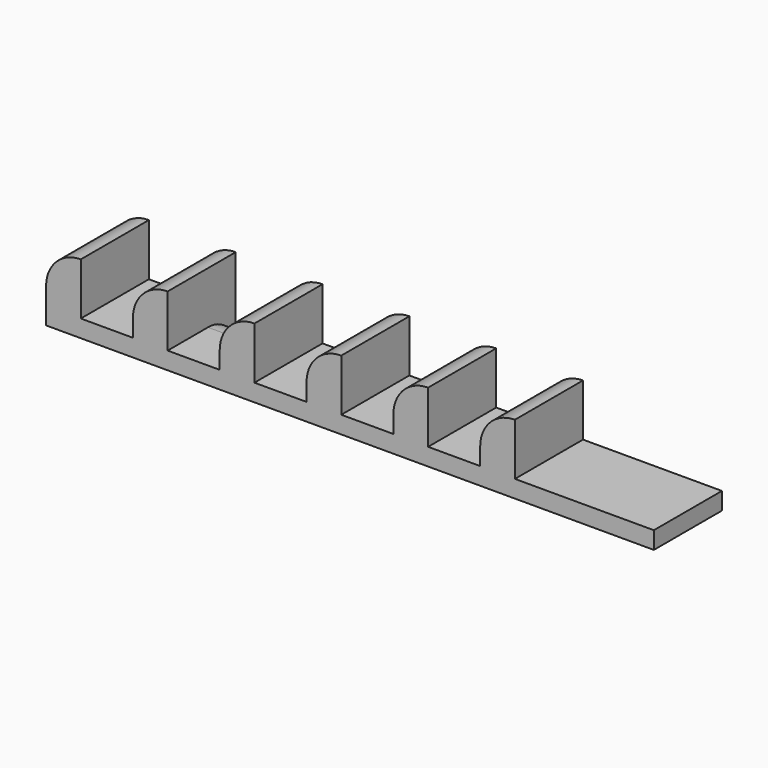
from build123d import *

# Parameters (mm, degrees)
F0_W        = 88.9
F0_H        = 12.446
F1_DEPTH    = 2.54
F2_W        = 5.08
F2_H        = 12.446
F3_DEPTH    = 7.62
F4_T1_DEPTH = 37.846
F4_T3_DEPTH = 7.62


# Not quite as in the source:
# - a fillet or chamfer that OpenCascade refuses, or shapes differently, is made with other operations: its cross-section is extruded or revolved along the edge and cut away or added


with BuildPart() as f1:
    # F0 (on Top) → F1 (new body)
    with BuildSketch(Plane.XY):
        with Locations((-4.0042309799, -31.983400695)):
            Rectangle(F0_W, F0_H)
    extrude(amount=F1_DEPTH)

    # F2 (on face) → F3 (join)
    with BuildSketch(Plane.XY.offset(2.54)):
        with Locations((-45.9142309799, -31.983400695)):
            Rectangle(F2_W, F2_H)
        with Locations((-33.2142309799, -31.983400695)):
            Rectangle(F2_W, F2_H)
        with Locations((-20.5142309799, -31.983400695)):
            Rectangle(F2_W, F2_H)
        with Locations((-7.8142309799, -31.983400695)):
            Rectangle(F2_W, F2_H)
        with Locations((4.8857690201, -31.983400695)):
            Rectangle(F2_W, F2_H)
        with Locations((17.5857690201, -31.983400695)):
            Rectangle(F2_W, F2_H)
    extrude(amount=F3_DEPTH)

    # F4: fillet of radius 5.08 on 7 edges, made by hand

    # F4_s2 → F4_t1 (cut)
    with BuildSketch(Plane.XZ.offset(13.060400695)):
        with BuildLine():
            ThreePointArc((-48.4542309799, 5.08), (-46.9663334283, 8.6721024484), (-43.3742309799, 10.16))
            Line((-43.3742309799, 10.16), (-48.4542309799, 10.16))
            Line((-48.4542309799, 10.16), (-48.4542309799, 5.08))
        make_face()
        with BuildLine():
            ThreePointArc((-30.6742309799, 10.16), (-34.2663334283, 8.6721024484), (-35.7542309799, 5.08))
            Line((-35.7542309799, 5.08), (-35.7542309799, 10.16))
            Line((-35.7542309799, 10.16), (-30.6742309799, 10.16))
        make_face()
        with BuildLine():
            ThreePointArc((-17.9742309799, 10.16), (-21.5663334283, 8.6721024484), (-23.0542309799, 5.08))
            Line((-23.0542309799, 5.08), (-23.0542309799, 10.16))
            Line((-23.0542309799, 10.16), (-17.9742309799, 10.16))
        make_face()
        with BuildLine():
            ThreePointArc((-5.2742309799, 10.16), (-8.8663334283, 8.6721024484), (-10.3542309799, 5.08))
            Line((-10.3542309799, 5.08), (-10.3542309799, 10.16))
            Line((-10.3542309799, 10.16), (-5.2742309799, 10.16))
        make_face()
        with BuildLine():
            ThreePointArc((7.4257690201, 10.16), (3.8336665717, 8.6721024484), (2.3457690201, 5.08))
            Line((2.3457690201, 5.08), (2.3457690201, 10.16))
            Line((2.3457690201, 10.16), (7.4257690201, 10.16))
        make_face()
        with BuildLine():
            ThreePointArc((20.1257690201, 10.16), (16.5336665717, 8.6721024484), (15.0457690201, 5.08))
            Line((15.0457690201, 5.08), (15.0457690201, 10.16))
            Line((15.0457690201, 10.16), (20.1257690201, 10.16))
        make_face()
    extrude(amount=F4_T1_DEPTH, mode=Mode.SUBTRACT)

    # F4_s4 → F4_t3 (cut)
    with BuildSketch(Plane.YZ.offset(-30.6742309799)):
        with BuildLine():
            ThreePointArc((-30.840400695, 2.54), (-27.2482982466, 1.0521024484), (-25.760400695, -2.54))
            Line((-25.760400695, -2.54), (-25.760400695, 2.54))
            Line((-25.760400695, 2.54), (-30.840400695, 2.54))
        make_face()
    extrude(amount=F4_T3_DEPTH, mode=Mode.SUBTRACT)


solid = f1.part
